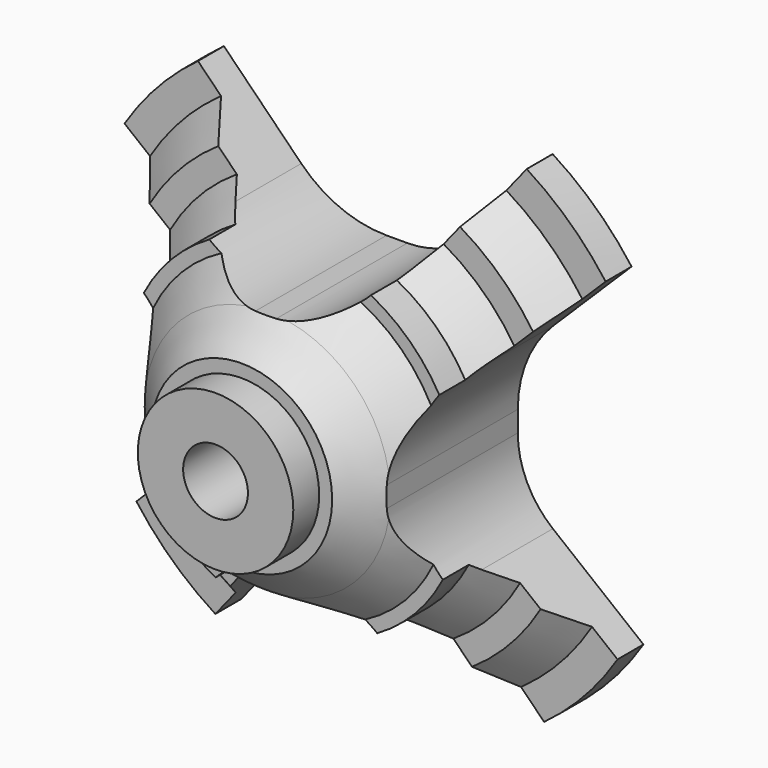
from build123d import *

# Parameters (mm, degrees)
F0_R      = 12
F0_R_2    = 5
F1_DEPTH  = 35
F0_R_3    = 19
F2_DEPTH  = 30
F0_R_4    = 26
F3_DEPTH  = 20
F0_R_5    = 40
F4_DEPTH  = 10
F0_R_6    = 45
F5_DEPTH  = 5
F9_SIZE   = 4.99999
F10_DEPTH = 50
F11_SIZE  = 4.99999
F13_DEPTH = 50
F14_R     = 18.5105769834
F15_R     = 14.4105910726
F16_ANGLE = 90
F17_ANGLE = 180
F18_ANGLE = 270


# Not quite as in the source:
# - a fillet or chamfer is up to 0.001 mm smaller than in the source, because OpenCascade refuses the exact size


with BuildPart() as f1:
    # F0 (on Front) → F1 (new body)
    with BuildSketch(Plane.XZ):
        Circle(F0_R)
        Circle(F0_R_2, mode=Mode.SUBTRACT)
    extrude(amount=F1_DEPTH)

    # F0 (on Front) → F2 (join)
    with BuildSketch(Plane.XZ):
        Circle(F0_R_3)
        Circle(F0_R, mode=Mode.SUBTRACT)
    extrude(amount=F2_DEPTH)

    # F0 (on Front) → F3 (join)
    with BuildSketch(Plane.XZ):
        Circle(F0_R_4)
        Circle(F0_R_3, mode=Mode.SUBTRACT)
    extrude(amount=F3_DEPTH)

    # F0 (on Front) → F4 (join)
    with BuildSketch(Plane.XZ):
        Circle(F0_R_5)
        Circle(F0_R_4, mode=Mode.SUBTRACT)
    extrude(amount=F4_DEPTH)

    # F0 (on Front) → F5 (join)
    with BuildSketch(Plane.XZ):
        Circle(F0_R_6)
        Circle(F0_R_5, mode=Mode.SUBTRACT)
    extrude(amount=F5_DEPTH)

    # F9 (size 5 in the source; OpenCascade refuses exactly that, so slightly less here)
    f9_edges = [f1.edges().sort_by_distance(p)[0] for p in [
        (-40, -10, 0),
        (-26, -10, 0),
    ]]
    chamfer(f9_edges, length=F9_SIZE)

    # F0 (on Front) → F10 (cut)
    with BuildSketch(Plane.XZ):
        Circle(F0_R_2)
    extrude(amount=-F10_DEPTH, mode=Mode.SUBTRACT)

    # F11 (size 5 in the source; OpenCascade refuses exactly that, so slightly less here)
    f11_edges = [f1.edges().sort_by_distance(p)[0] for p in [
        (-19, -20, 0),
        (19, -25, 0),
        (-19, -30, 0),
    ]]
    chamfer(f11_edges, length=F11_SIZE)


with BuildPart() as f13:
    # F12 (on Front) → F13 (new body)
    with BuildSketch(Plane.XZ):
        Polygon((30.8662448078, 46.592772007), (-38.6121459305, 48.2358410954), (-9.3319928274, 18.6549890786), (8.5259051993, 18.6549890786), align=None)
    extrude(amount=F13_DEPTH)

    # F14
    f14_edges = [f13.edges().sort_by_distance(p)[0] for p in [
        (-9.331993, -25, 18.654989),
    ]]
    fillet(f14_edges, radius=F14_R)

    # F15
    f15_edges = [f13.edges().sort_by_distance(p)[0] for p in [
        (8.525905, -25, 18.654989),
    ]]
    fillet(f15_edges, radius=F15_R)


with BuildPart() as f16_1:
    # F16: copy of F13
    add(f13.part.rotate(Axis((0, -35.1110678166, 0), (0, 1, 0)), F16_ANGLE))


with BuildPart() as f17_1:
    # F17: copy of F13
    add(f13.part.rotate(Axis((0, -20.7477975637, 0), (0, 1, 0)), F17_ANGLE))


with BuildPart() as f18_1:
    # F18: copy of F13
    add(f13.part.rotate(Axis((0, -17.8390480578, 0), (0, 1, 0)), F18_ANGLE))


with BuildPart() as f1_1:
    add(f1.part)

    # F19: cut F13
    add(f13.part, mode=Mode.SUBTRACT)

    # F20: cut F17_1
    add(f17_1.part, mode=Mode.SUBTRACT)

    # F21: cut F16_1
    add(f16_1.part, mode=Mode.SUBTRACT)

    # F22: cut F18_1
    add(f18_1.part, mode=Mode.SUBTRACT)


solid = f1_1.part
